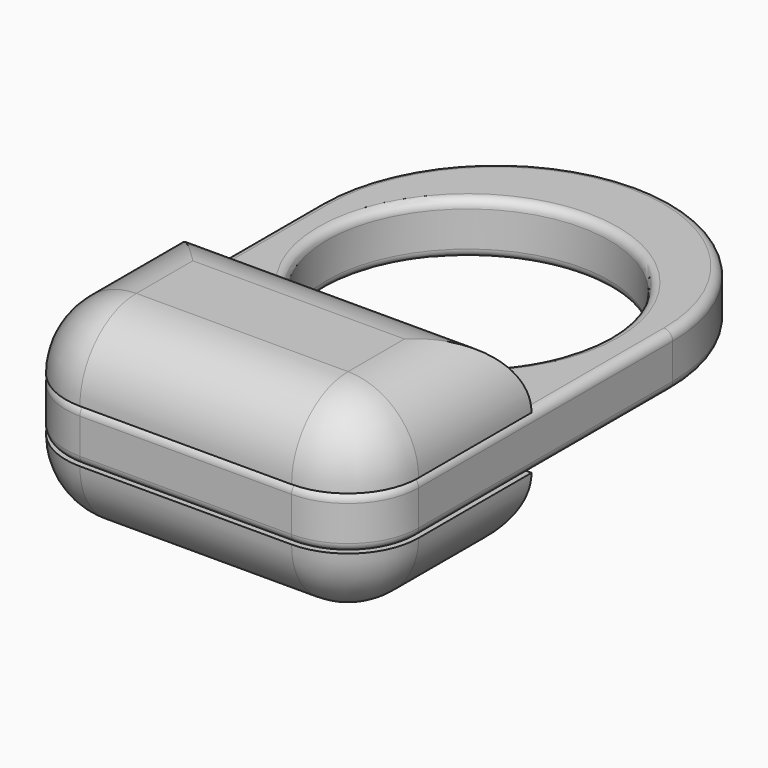
from build123d import *

# Parameters (mm, degrees)
F0_R     = 12.7
F1_DEPTH = 4.7625
F3_DEPTH = 6.35
F5_DEPTH = 6.35
F6_R     = 6.34999
F6_2_R   = 6.34999
F7_R     = 0.79375


# Not quite as in the source:
# - a fillet or chamfer is up to 0.001 mm smaller than in the source, because OpenCascade refuses the exact size


with BuildPart() as f1:
    # F0 (on Top) → F1 (new body)
    with BuildSketch(Plane.XY):
        with BuildLine():
            Line((-9.525, -25.4), (9.525, -25.4))
            ThreePointArc((9.525, -25.4), (14.0151280605, -23.5401280605), (15.875, -19.05))
            Line((15.875, -19.05), (15.875, 9.525))
            ThreePointArc((15.875, 9.525), (0, 25.4), (-15.875, 9.525))
            Line((-15.875, 9.525), (-15.875, -19.05))
            ThreePointArc((-15.875, -19.05), (-14.0151280605, -23.5401280605), (-9.525, -25.4))
        make_face()
        with Locations((0, 6.35)):
            Circle(F0_R, mode=Mode.SUBTRACT)
    extrude(amount=F1_DEPTH)

    # F7
    f7_edges = [f1.edges().sort_by_distance(p)[0] for p in [
        (-15.875, -4.7625, 4.7625),
        (-14.015128, -23.540128, 4.7625),
        (0, -25.4, 4.7625),
        (14.015128, -23.540128, 4.7625),
        (15.875, -4.7625, 4.7625),
        (0, 25.4, 4.7625),
        (-12.7, 6.35, 4.7625),
        (-15.875, -4.7625, 0),
        (-14.015128, -23.540128, 0),
        (0, -25.4, 0),
        (14.015128, -23.540128, 0),
        (15.875, -4.7625, 0),
        (0, 25.4, 0),
        (-12.7, 6.35, 0),
    ]]
    fillet(f7_edges, radius=F7_R)


with BuildPart() as f3:
    # F2 (on face) → F3 (new body)
    with BuildSketch(Plane.XY.offset(4.7625)):
        with BuildLine():
            Line((15.875, -6.35), (0, -6.35))
            Line((0, -6.35), (-15.875, -6.35))
            Line((-15.875, -6.35), (-15.875, -19.05))
            ThreePointArc((-15.875, -19.05), (-14.0151280605, -23.5401280605), (-9.525, -25.4))
            Line((-9.525, -25.4), (9.525, -25.4))
            ThreePointArc((9.525, -25.4), (14.0151280605, -23.5401280605), (15.875, -19.05))
            Line((15.875, -19.05), (15.875, -6.35))
        make_face()
    extrude(amount=F3_DEPTH)

    # F6#2 (radius 6.35 in the source; OpenCascade refuses exactly that, so slightly less here)
    f6_2_edges = [f3.edges().sort_by_distance(p)[0] for p in [
        (0, -6.35, 11.1125),
        (-15.875, -12.7, 11.1125),
        (-14.015128, -23.540128, 11.1125),
        (0, -25.4, 11.1125),
        (14.015128, -23.540128, 11.1125),
        (15.875, -12.7, 11.1125),
    ]]
    fillet(f6_2_edges, radius=F6_2_R)


with BuildPart() as f5:
    # F4 (on face) → F5 (new body)
    with BuildSketch(Plane(origin=(0, 0, 0), x_dir=(1, 0, 0), z_dir=(0, 0, -1))):
        with BuildLine():
            Line((-15.875, 6.35), (0, 6.35))
            Line((0, 6.35), (15.875, 6.35))
            Line((15.875, 6.35), (15.875, 19.05))
            ThreePointArc((15.875, 19.05), (14.0151280605, 23.5401280605), (9.525, 25.4))
            Line((9.525, 25.4), (-9.525, 25.4))
            ThreePointArc((-9.525, 25.4), (-14.0151280605, 23.5401280605), (-15.875, 19.05))
            Line((-15.875, 19.05), (-15.875, 6.35))
        make_face()
    extrude(amount=F5_DEPTH)

    # F6 (radius 6.35 in the source; OpenCascade refuses exactly that, so slightly less here)
    f6_edges = [f5.edges().sort_by_distance(p)[0] for p in [
        (-15.875, -12.7, -6.35),
        (0, -6.35, -6.35),
        (15.875, -12.7, -6.35),
        (14.015128, -23.540128, -6.35),
        (0, -25.4, -6.35),
        (-14.015128, -23.540128, -6.35),
    ]]
    fillet(f6_edges, radius=F6_R)


solid = Compound([f1.part, f3.part, f5.part])
